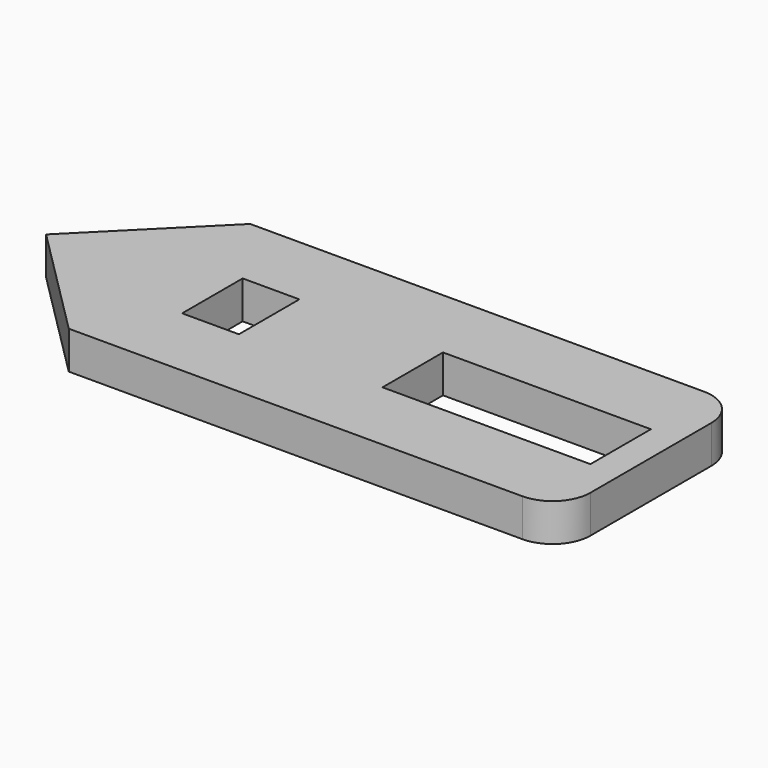
from build123d import *

# Parameters (mm, degrees)
F0_W     = 80
F0_H     = 30
F1_DEPTH = 5
F2_W     = 7.5
F2_H     = 10
F3_DEPTH = 25
F4_W     = 27.5
F4_H     = 10
F5_DEPTH = 5
F6_SIZE  = 14.99999
F7_R     = 5


# Not quite as in the source:
# - a fillet or chamfer is up to 0.001 mm smaller than in the source, because OpenCascade refuses the exact size


with BuildPart() as f1:
    # F0 (on Top) → F1 (new body)
    with BuildSketch(Plane.XY):
        with Locations((3.5, 0)):
            Rectangle(F0_W, F0_H)
    extrude(amount=F1_DEPTH)

    # F2 (on face) → F3 (cut)
    with BuildSketch(Plane.XY.offset(5)):
        with Locations((-10.75, 0)):
            Rectangle(F2_W, F2_H)
    extrude(amount=-F3_DEPTH, mode=Mode.SUBTRACT)

    # F4 (on face) → F5 (cut)
    with BuildSketch(Plane.XY.offset(5)):
        with Locations((25.75, 0)):
            Rectangle(F4_W, F4_H)
    extrude(amount=-F5_DEPTH, mode=Mode.SUBTRACT)

    # F6 (size 15 in the source; OpenCascade refuses exactly that, so slightly less here)
    f6_edges = [f1.edges().sort_by_distance(p)[0] for p in [
        (-36.5, -15, 2.5),
        (-36.5, 15, 2.5),
    ]]
    chamfer(f6_edges, length=F6_SIZE)

    # F7
    f7_edges = [f1.edges().sort_by_distance(p)[0] for p in [
        (43.5, -15, 2.5),
        (43.5, 15, 2.5),
    ]]
    fillet(f7_edges, radius=F7_R)


solid = f1.part
